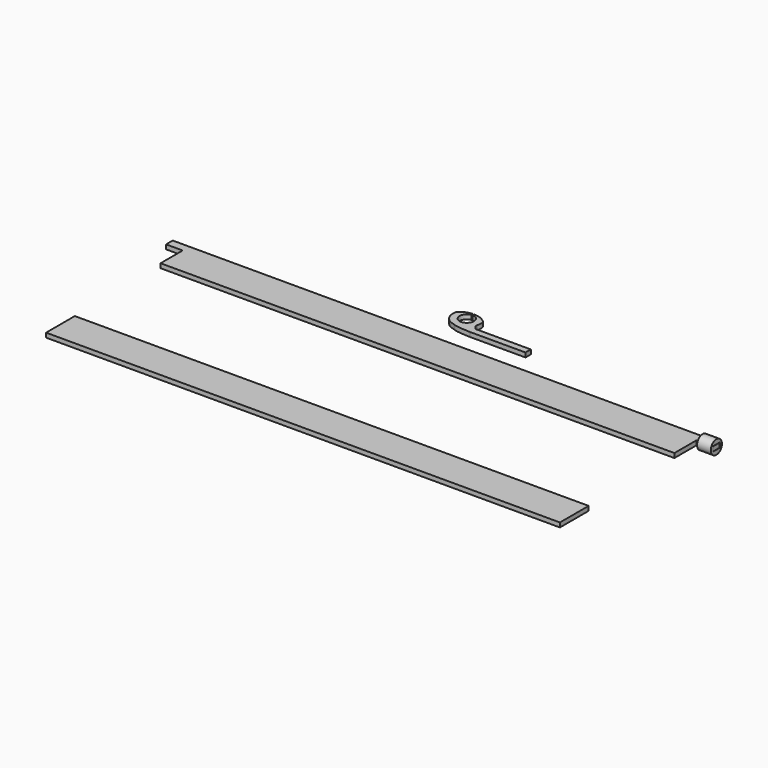
from build123d import *

# Parameters (mm, degrees)
F0_W     = 30
F0_H     = 15
F1_DEPTH = 8
F0_W_2   = 930
F0_H_2   = 65
F2_R     = 12.5
F2_W     = 15.8
F2_H     = 8.8
F3_DEPTH = 25
F5_DEPTH = 8


with BuildPart() as f1:
    # F0 (on Top) → F1 (new body)
    with BuildSketch(Plane.XY):
        with Locations((480, 0)):
            Rectangle(F0_W, F0_H)
        Polygon((465, -7.5), (465, 7.5), (-465, 7.5), (-465, -7.5), (-465, -57.5), (465, -57.5), align=None)
        with Locations((-480, 0)):
            Rectangle(F0_W, F0_H)
    extrude(amount=F1_DEPTH)


with BuildPart() as f1b:
    # F0 (on Top) → F1, piece 2 (new body)
    with BuildSketch(Plane.XY):
        with Locations((6.3626134396, -291.9821131229)):
            Rectangle(F0_W_2, F0_H_2)
    extrude(amount=F1_DEPTH)


with BuildPart() as f3:
    # F2 (on face) → F3 (new body)
    with BuildSketch(Plane.YZ.offset(495)):
        with Locations((0, 4)):
            Circle(F2_R)
        with Locations((0, 4)):
            Rectangle(F2_W, F2_H, mode=Mode.SUBTRACT)
    extrude(amount=-F3_DEPTH)


with BuildPart() as f5:
    # F4 (on Top) → F5 (new body)
    with BuildSketch(Plane.XY):
        with BuildLine():
            Line((108.3438670263, 51.3812564313), (108.3438670263, 63.3812564313))
            Line((108.3438670263, 63.3812564313), (8.3438670263, 63.3812564313))
            add(Edge.make_bspline(
                [(8.3438670263, 63.3812564313), (5.3670516377, 66.7041790393), (2.4126594236, 70.0207141177), (2.5014199346, 72.6916081624)],
                knots=[0, 0, 0, 0, 0.5599704127, 0.5599704127, 0.5599704127, 0.5599704127], degree=3))
            add(Edge.make_bspline(
                [(2.5014199346, 72.6916081624), (2.5224130391, 73.3233120261), (2.7136366909, 73.9188994552), (3.0243427489, 74.4891023385)],
                knots=[0.5599704127, 0.5599704127, 0.5599704127, 0.5599704127, 0.6924112611, 0.6924112611, 0.6924112611, 0.6924112611], degree=3))
            ThreePointArc((3.0243427489, 74.4891023385), (3.7708143316, 81.0199999582), (2.7891735817, 87.5197095656))
            ThreePointArc((2.7891735817, 87.5197095656), (-8.1359373234, 94.5418353751), (-20.8645367822, 97.1207993121))
            Line((-20.8645367822, 97.1207993121), (-20.8645367822, 93.5638856829))
            ThreePointArc((-20.8645367822, 93.5638856829), (-20.4989886716, 67.5891823606), (-23.0328720233, 93.4425820067))
            Line((-23.0328720233, 93.4425820067), (-23.0328720233, 97.0847913286))
            ThreePointArc((-23.0328720233, 97.0847913286), (-34.8898145719, 94.420179027), (-45.1322930826, 87.8796225313))
            ThreePointArc((-45.1322930826, 87.8796225313), (-42.3366661495, 67.1785019342), (-24.8017338771, 55.8260539988))
            add(Edge.make_bspline(
                [(8.3438670263, 51.3812564313), (-5.3752977401, 51.7728589475), (-18.1325646639, 52.2421691312), (-24.8017338771, 55.8260539988)],
                knots=[0, 0, 0, 0, 0.6343210063, 0.6343210063, 0.6343210063, 0.6343210063], degree=3))
            Line((8.3438670263, 51.3812564313), (108.3438670263, 51.3812564313))
        make_face()
        with BuildLine():
            add(Edge.make_bspline(
                [(2.5014199346, 72.6916081624), (2.5224130391, 73.3233120261), (2.7136366909, 73.9188994552), (3.0243427489, 74.4891023385)],
                knots=[0.5599704127, 0.5599704127, 0.5599704127, 0.5599704127, 0.6924112611, 0.6924112611, 0.6924112611, 0.6924112611], degree=3))
            ThreePointArc((2.5014199346, 72.6916081624), (2.7797119065, 73.5854589418), (3.0243427489, 74.4891023385))
        make_face()
    extrude(amount=F5_DEPTH)


solid = Compound([f1.part, f1b.part, f3.part, f5.part])
